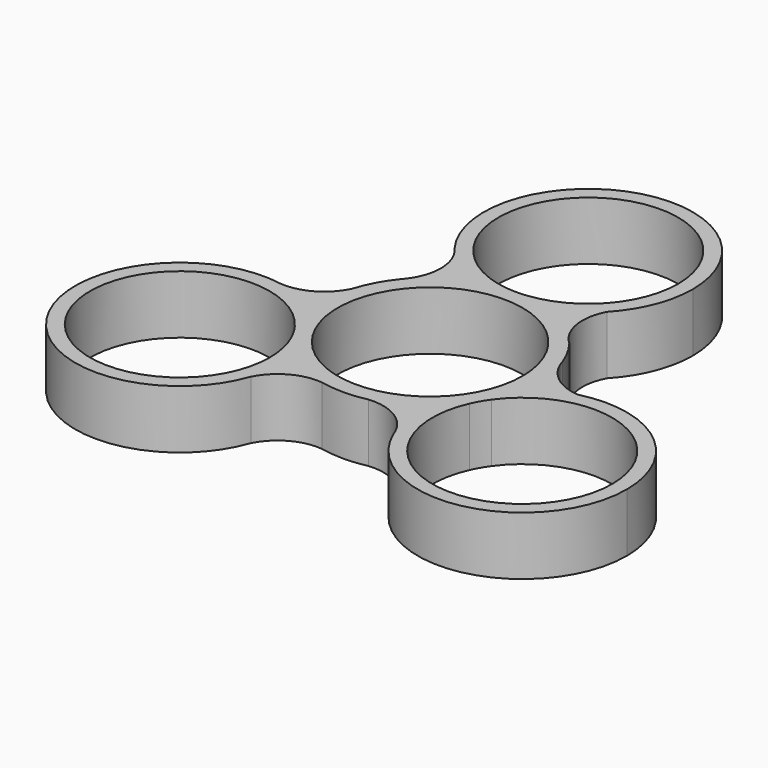
from build123d import *

# Parameters (mm, degrees)
F0_R     = 11.05
F1_DEPTH = 7


with BuildPart() as f1:
    # F0 (on Top) → F1 (new body)
    with BuildSketch(Plane.XY):
        with BuildLine():
            ThreePointArc((12.4036553845, 3.8922144215), (12.2588680886, 4.2668950825), (12.1397217876, 4.650500502))
            ThreePointArc((12.1397217876, 4.650500502), (11.3509584551, 6.3368558568), (10.3294036233, 7.8932515979))
            ThreePointArc((10.3294036233, 7.8932515979), (9.8245761866, 8.414561478), (9.3870501636, 8.9935137308))
            ThreePointArc((9.3870501636, 8.9935137308), (7.2468764963, 10.7927188904), (4.7714819389, 12.092682089))
            ThreePointArc((4.7714819389, 12.092682089), (0, 11.1461646855), (-4.7714819389, 12.092682089))
            ThreePointArc((-4.7714819389, 12.092682089), (-7.5081755961, 10.6126009639), (-9.8148092936, 8.5246418417))
            ThreePointArc((-9.8148092936, 8.5246418417), (-9.9218729104, 8.3943935706), (-10.0325882839, 8.2672348658))
            ThreePointArc((-10.0325882839, 8.2672348658), (-11.4424495934, 6.1701172844), (-12.419961597, 3.8398637906))
            ThreePointArc((-12.419961597, 3.8398637906), (-12.9624394617, 0.9875035204), (-12.8583108585, -1.9141164717))
            ThreePointArc((-12.8583108585, -1.9141164717), (-9.6528617724, -5.5730823427), (-8.0868289195, -10.1785656173))
            ThreePointArc((-8.0868289195, -10.1785656173), (-5.5850066858, -11.7391524532), (-2.7958525219, -12.695794921))
            ThreePointArc((-2.7958525219, -12.695794921), (0.0017952144, -12.999999876), (2.7993588265, -12.6950222592))
            ThreePointArc((2.7993588265, -12.6950222592), (5.5866277322, -11.7383810886), (8.0868289195, -10.1785656173))
            ThreePointArc((8.0868289195, -10.1785656173), (9.6528617724, -5.5730823427), (12.8583108585, -1.9141164717))
            ThreePointArc((12.8583108585, -1.9141164717), (12.9645293235, -0.9596767268), (13, 0))
            ThreePointArc((13, 0), (12.8500490271, 1.9688169038), (12.4036553845, 3.8922144215))
        make_face()
        Circle(F0_R, mode=Mode.SUBTRACT)
        with BuildLine():
            ThreePointArc((17.4129621968, 0.2952691949), (14.4052350934, 1.3931332806), (12.4036553845, 3.8922144215))
            ThreePointArc((12.4036553845, 3.8922144215), (12.8500490271, 1.9688169038), (13, 0))
            ThreePointArc((13, 0), (12.9645293235, -0.9596767268), (12.8583108585, -1.9141164717))
            ThreePointArc((12.8583108585, -1.9141164717), (15.0226216268, -0.5764432777), (17.4129621968, 0.2952691949))
        make_face()
        with BuildLine():
            ThreePointArc((4.7714819389, 12.092682089), (7.2468764963, 10.7927188904), (9.3870501636, 8.9935137308))
            ThreePointArc((9.3870501636, 8.9935137308), (8.402604273, 11.9865844679), (9.0866097244, 15.0622539383))
            ThreePointArc((9.0866097244, 15.0622539383), (7.0863435832, 13.3488963768), (4.7714819389, 12.092682089))
        make_face()
        with BuildLine():
            ThreePointArc((32.9781793197, -11.8230823427), (28.1572022381, -1.9598877782), (17.4129621968, 0.2952691949))
            ThreePointArc((17.4129621968, 0.2952691949), (15.0226216268, -0.5764432777), (12.8583108585, -1.9141164717))
            ThreePointArc((12.8583108585, -1.9141164717), (12.4453302152, -3.7568278952), (11.7697355483, -5.5202649505))
            ThreePointArc((11.7697355483, -5.5202649505), (23.7907862581, -1.5961993733), (31.2281793197, -11.8230823427))
            ThreePointArc((31.2281793197, -11.8230823427), (18.2335395964, -22.3361262651), (10.6655574569, -7.4327575054))
            ThreePointArc((10.6655574569, -7.4327575054), (9.4761735025, -8.8995581772), (8.0868289195, -10.1785656173))
            ThreePointArc((8.0868289195, -10.1785656173), (8.05547786, -13.2110623297), (8.7553384731, -16.161861259))
            ThreePointArc((8.7553384731, -16.161861259), (8.8665325035, -16.4239751001), (8.9650446915, -16.6911138785))
            ThreePointArc((8.9650446915, -16.6911138785), (22.9617067654, -24.0738819667), (32.9781793197, -11.8230823427))
        make_face()
        with BuildLine():
            ThreePointArc((-4.7714819389, 12.092682089), (0, 11.1461646855), (4.7714819389, 12.092682089))
            ThreePointArc((4.7714819389, 12.092682089), (2.9691567127, 12.6563860725), (1.1041780914, 12.9530224559))
            ThreePointArc((1.1041780914, 12.9530224559), (0, 12.8961646855), (-1.1041780914, 12.9530224559))
            ThreePointArc((-1.1041780914, 12.9530224559), (-2.9691567127, 12.6563860725), (-4.7714819389, 12.092682089))
        make_face()
        with BuildLine():
            ThreePointArc((1.1041780914, 12.9530224559), (2.9691567127, 12.6563860725), (4.7714819389, 12.092682089))
            ThreePointArc((4.7714819389, 12.092682089), (7.0863435832, 13.3488963768), (9.0866097244, 15.0622539383))
            ThreePointArc((9.0866097244, 15.0622539383), (11.6153480696, 19.027324006), (12.5, 23.6461646855))
            ThreePointArc((12.5, 23.6461646855), (-3.8986180344, 35.5226446952), (-10.0681243875, 16.2378672213))
            ThreePointArc((-10.0681243875, 16.2378672213), (-9.794102473, 15.9150690623), (-9.5437602938, 15.5735790121))
            ThreePointArc((-9.5437602938, 15.5735790121), (-7.3661863194, 13.5471895341), (-4.7714819389, 12.092682089))
            ThreePointArc((-4.7714819389, 12.092682089), (-2.9691567127, 12.6563860725), (-1.1041780914, 12.9530224559))
            ThreePointArc((-1.1041780914, 12.9530224559), (-7.2004369839, 31.6284079317), (10.75, 23.6461646855))
            ThreePointArc((10.75, 23.6461646855), (7.9822432462, 16.4457277016), (1.1041780914, 12.9530224559))
        make_face()
        with BuildLine():
            ThreePointArc((11.7697355483, -5.5202649505), (12.4453302152, -3.7568278952), (12.8583108585, -1.9141164717))
            ThreePointArc((12.8583108585, -1.9141164717), (9.6528617724, -5.5730823427), (8.0868289195, -10.1785656173))
            ThreePointArc((8.0868289195, -10.1785656173), (9.4761735025, -8.8995581772), (10.6655574569, -7.4327575054))
            ThreePointArc((10.6655574569, -7.4327575054), (11.168406229, -6.4480823427), (11.7697355483, -5.5202649505))
        make_face()
        with BuildLine():
            ThreePointArc((-9.8148092936, 8.5246418417), (-7.5081755961, 10.6126009639), (-4.7714819389, 12.092682089))
            ThreePointArc((-4.7714819389, 12.092682089), (-7.3661863194, 13.5471895341), (-9.5437602938, 15.5735790121))
            ThreePointArc((-9.5437602938, 15.5735790121), (-8.5203205537, 12.0045453967), (-9.8148092936, 8.5246418417))
        make_face()
        with BuildLine():
            ThreePointArc((8.7553384731, -16.161861259), (8.05547786, -13.2110623297), (8.0868289195, -10.1785656173))
            ThreePointArc((8.0868289195, -10.1785656173), (5.5866277322, -11.7383810886), (2.7993588265, -12.6950222592))
            ThreePointArc((2.7993588265, -12.6950222592), (6.3311702253, -13.4769842407), (8.7553384731, -16.161861259))
        make_face()
        with BuildLine():
            ThreePointArc((-8.6738467532, -15.9349836863), (-6.2358648809, -13.4062219399), (-2.7958525219, -12.695794921))
            ThreePointArc((-2.7958525219, -12.695794921), (-5.5850066858, -11.7391524532), (-8.0868289195, -10.1785656173))
            ThreePointArc((-8.0868289195, -10.1785656173), (-8.0053712958, -10.9990313741), (-7.9781793197, -11.8230823427))
            ThreePointArc((-7.9781793197, -11.8230823427), (-8.1533231931, -13.9082493527), (-8.6738467532, -15.9349836863))
        make_face()
        with BuildLine():
            ThreePointArc((-12.8583108585, -1.9141164717), (-12.9624394617, 0.9875035204), (-12.419961597, 3.8398637906))
            ThreePointArc((-12.419961597, 3.8398637906), (-14.8010494837, 1.2584054136), (-18.2237650289, 0.4719416997))
            ThreePointArc((-18.2237650289, 0.4719416997), (-15.3989388877, -0.4015536958), (-12.8583108585, -1.9141164717))
        make_face()
        with BuildLine():
            ThreePointArc((-7.9781793197, -11.8230823427), (-8.0053712958, -10.9990313741), (-8.0868289195, -10.1785656173))
            ThreePointArc((-8.0868289195, -10.1785656173), (-9.4761735025, -8.8995581772), (-10.6655574569, -7.4327575054))
            ThreePointArc((-10.6655574569, -7.4327575054), (-9.9651353974, -9.5784426194), (-9.7281793197, -11.8230823427))
            ThreePointArc((-9.7281793197, -11.8230823427), (-30.7050622892, -15.1356892812), (-11.7697355483, -5.5202649505))
            ThreePointArc((-11.7697355483, -5.5202649505), (-12.4453302152, -3.7568278952), (-12.8583108585, -1.9141164717))
            ThreePointArc((-12.8583108585, -1.9141164717), (-15.3989388877, -0.4015536958), (-18.2237650289, 0.4719416997))
            ThreePointArc((-18.2237650289, 0.4719416997), (-31.281368245, -18.1112544972), (-8.6738467532, -15.9349836863))
            ThreePointArc((-8.6738467532, -15.9349836863), (-8.1533231931, -13.9082493527), (-7.9781793197, -11.8230823427))
        make_face()
        with BuildLine():
            ThreePointArc((-10.6655574569, -7.4327575054), (-9.4761735025, -8.8995581772), (-8.0868289195, -10.1785656173))
            ThreePointArc((-8.0868289195, -10.1785656173), (-9.6528617724, -5.5730823427), (-12.8583108585, -1.9141164717))
            ThreePointArc((-12.8583108585, -1.9141164717), (-12.4453302152, -3.7568278952), (-11.7697355483, -5.5202649505))
            ThreePointArc((-11.7697355483, -5.5202649505), (-11.168406229, -6.4480823427), (-10.6655574569, -7.4327575054))
        make_face()
    extrude(amount=F1_DEPTH)


solid = f1.part
